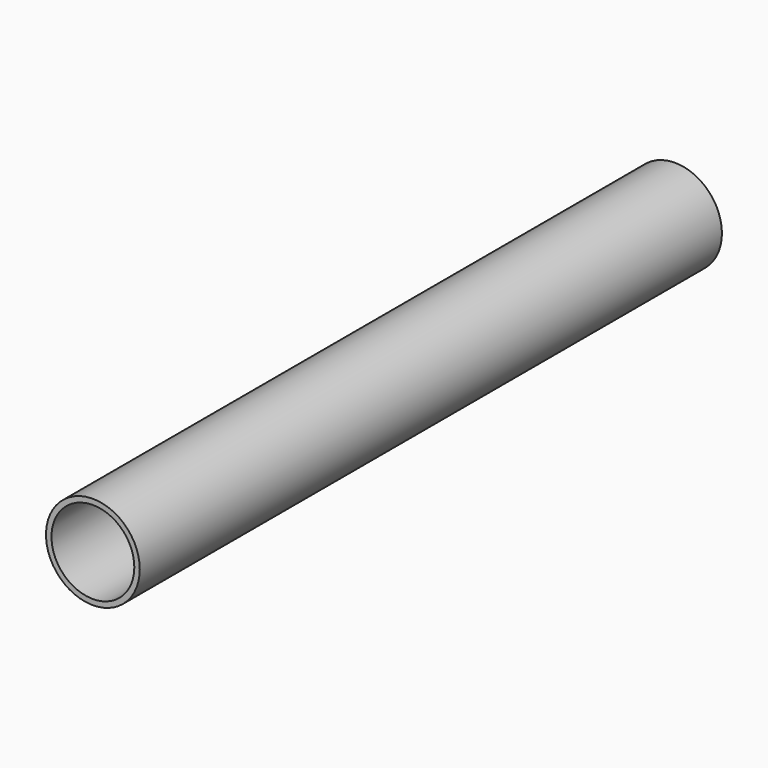
from build123d import *

# Parameters (mm, degrees)
F0_R     = 10.795
F0_R_2   = 9.5377
F1_DEPTH = 165.1
F2_R     = 10.795
F3_DEPTH = 2.42878


# Not quite as in the source:
# - a feature names something its author has since deleted; it is built from what else it names


with BuildPart() as f1:
    # F0 (on Front) → F1 (new body)
    with BuildSketch(Plane.XZ):
        Circle(F0_R)
        Circle(F0_R_2, mode=Mode.SUBTRACT)
    extrude(amount=F1_DEPTH)

    # F2 (on Front) → F3 (join)
    with BuildSketch(Plane.XZ):
        Circle(F2_R)
    extrude(amount=-F3_DEPTH)


solid = f1.part
